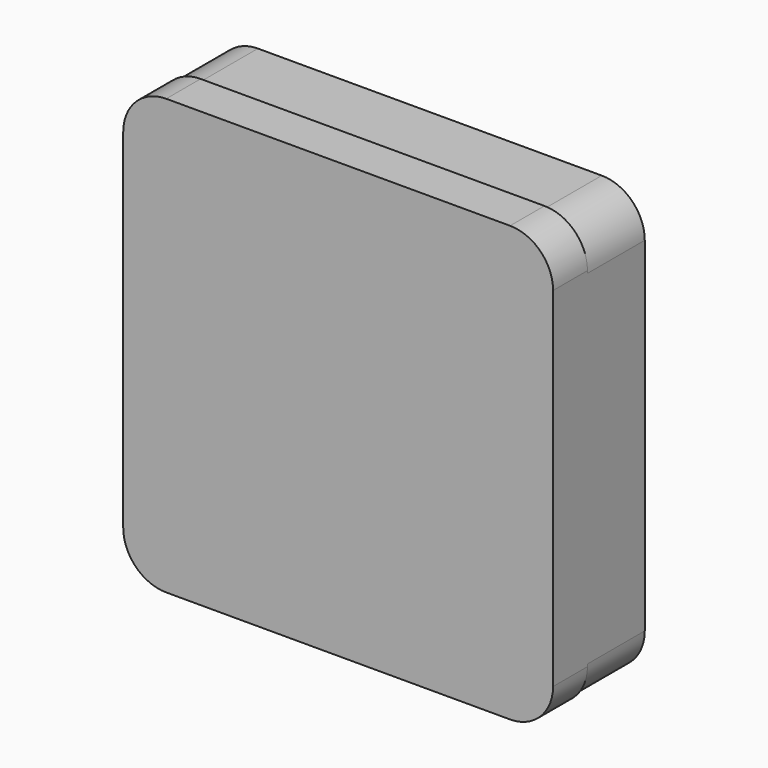
from build123d import *

# Parameters (mm, degrees)
F1_DEPTH = 12.7
F3_D     = 11.3284
F4_R     = 7.62
F5_W     = 76.2
F5_H     = 77.0487710834
F6_DEPTH = 7.62
F7_R     = 7.62


# Not quite as in the source:
# - a feature names something its author has since deleted; it is built from what else it names


with BuildPart() as f1:
    # F0 (on Front) → F1 (new body)
    with BuildSketch(Plane.XZ):
        Polygon((-38.1, -38.1), (38.1, -38.1), (38.1, -30.48), (38.1, 38.1), (-38.1, 38.1), align=None)
    extrude(amount=F1_DEPTH)

    # F3 (through all)
    with Locations(Plane.XZ.offset(12.7)):
        with Locations((-29.1592, 29.1592), (-14.5796, 29.1592), (0, 29.1592), (14.5796, 29.1592), (29.1592, 29.1592), (29.1592, 14.5796), (29.1592, 0), (29.1592, -14.5796), (29.1592, -29.1592), (14.5796, -29.1592), (14.5796, -14.5796), (14.5796, 0), (14.5796, 14.5796), (0, 14.5796), (0, 0), (0, -14.5796), (0, -29.1592), (-14.5796, -29.1592), (-14.5796, -14.5796), (-14.5796, 0), (-14.5796, 14.5796), (-29.1592, 14.5796), (-29.1592, 0), (-29.1592, -14.5796), (-29.1592, -29.1592)):
            Hole(F3_D / 2)

    # F4
    f4_edges = [f1.edges().sort_by_distance(p)[0] for p in [
        (-38.1, -6.35, 38.1),
        (38.1, -6.35, 38.1),
        (38.1, -6.35, -38.1),
        (-38.1, -6.35, -38.1),
    ]]
    fillet(f4_edges, radius=F4_R)

    # F5 (on face) → F6 (join)
    with BuildSketch(Plane.XZ.offset(12.7)):
        Rectangle(F5_W, F5_H)
    extrude(amount=F6_DEPTH)

    # F7
    f7_edges = [f1.edges().sort_by_distance(p)[0] for p in [
        (-38.1, -16.51, 38.524386),
        (38.1, -16.51, 38.524386),
        (38.1, -16.51, -38.524386),
        (-38.1, -16.51, -38.524386),
    ]]
    fillet(f7_edges, radius=F7_R)


solid = f1.part
